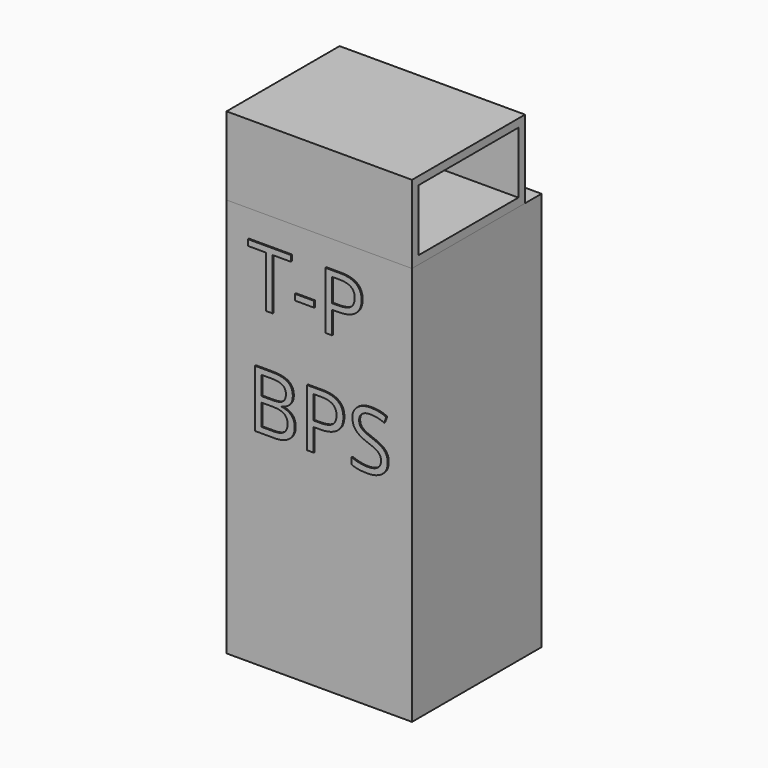
from build123d import *

# Parameters (mm, degrees)
F0_W         = 917.575
F0_H         = 800.735
F1_DEPTH     = 1974.85
F2_TEXT_SIZE = 397.3212507036
F3_DEPTH     = 6.35
F4_W         = 917.575
F4_H         = 800.735
F5_DEPTH     = 508
F6_W         = 718.185
F6_H         = 304.8
F7_DEPTH     = 1155.7
F8_DEPTH     = 121.92
F9_DEPTH     = 101.6
F10_DEPTH    = 101.6


# Not quite as in the source:
# - Text() gives the source's letters only with a copy of the font that has no kerning and outlines rounded to 1/6400 em; it was checked with that copy


with BuildPart() as f1:
    # F0 (on Top) → F1 (new body)
    with BuildSketch(Plane.XY):
        with Locations((458.7875, -400.3675)):
            Rectangle(F0_W, F0_H)
    extrude(amount=F1_DEPTH)

    # F2 (on face) → F3 (join)
    with BuildSketch(Plane.XZ.offset(800.735)):
        with Locations((106.8899855018, 1559.1375827789)):
            Text('T-P', F2_TEXT_SIZE, font='Open Sans', text_align=(TextAlign.LEFT, TextAlign.BOTTOM))
        with Locations((106.8899855018, 1018.780681822)):
            Text('BPS', F2_TEXT_SIZE, font='Open Sans', text_align=(TextAlign.LEFT, TextAlign.BOTTOM))
    extrude(amount=F3_DEPTH)


with BuildPart() as f5:
    # F4 (on face) → F5 (new body)
    with BuildSketch(Plane.XY.offset(1974.85)):
        with Locations((458.7875, -400.3675)):
            Rectangle(F4_W, F4_H)
    extrude(amount=F5_DEPTH)

    # F6 (on face) → F7 (cut)
    with BuildSketch(Plane.YZ.offset(917.575)):
        with Locations((-400.3675, 2168.525)):
            Rectangle(F6_W, F6_H)
    extrude(amount=-F7_DEPTH, mode=Mode.SUBTRACT)

    # F8 (cut): a face of the model
    f8_faces = [f5.faces().sort_by_distance(p)[0] for p in [
        (458.7875, -400.3675, 2482.85),
    ]]
    extrude(f8_faces, amount=-F8_DEPTH, mode=Mode.SUBTRACT)

    # F9 (add): a face of the model
    f9_faces = [f5.faces().sort_by_distance(p)[0] for p in [
        (458.7875, -41.275, 2168.525),
    ]]
    extrude(f9_faces, amount=F9_DEPTH)

    # F10 (cut): a face of the model
    f10_faces = [f5.faces().sort_by_distance(p)[0] for p in [
        (458.7875, 0, 2167.89),
    ]]
    extrude(f10_faces, amount=-F10_DEPTH, mode=Mode.SUBTRACT)


solid = Compound([f1.part, f5.part])
